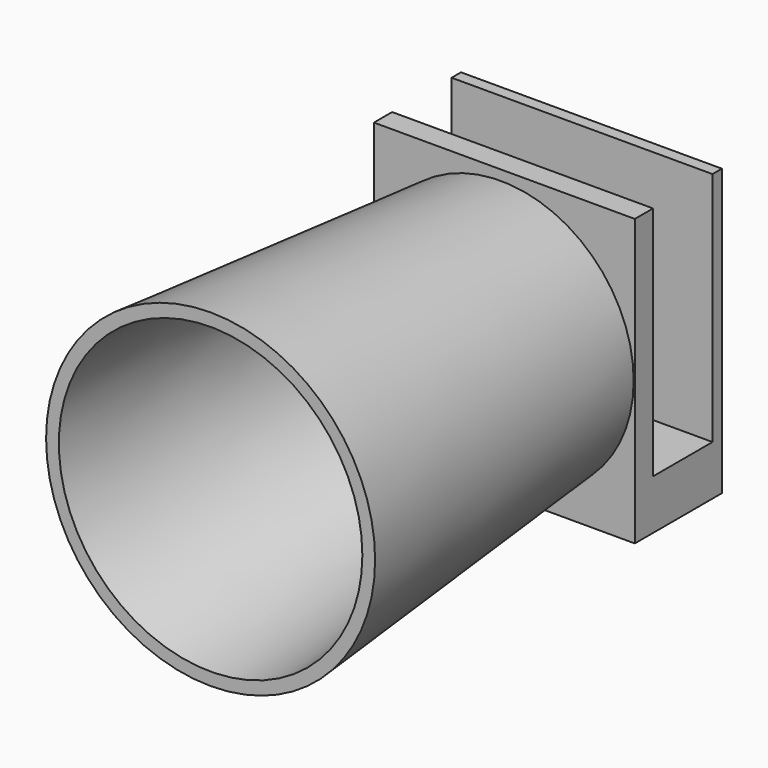
from build123d import *

# Parameters (mm, degrees)
F0_W     = 71.9023197889
F0_H     = 78.7298418581
F1_DEPTH = 30
F2_R     = 36.5885181047
F3_DEPTH = 100
F3_TAPER = -5
F4_T     = -3.5
F5_W     = 71.9023197889
F5_H     = 20.4825603869
F6_DEPTH = 65
F7_R     = 2.9162112623
F8_DEPTH = 0.7


# Not quite as in the source:
# - a feature names something its author has since deleted; it is built from what else it names


with BuildPart() as f1:
    # F0 (on Front) → F1 (new body)
    with BuildSketch(Plane.XZ):
        with Locations((0.9601190686, -0.0165458769)):
            Rectangle(F0_W, F0_H)
    extrude(amount=-F1_DEPTH)

    # F5 (on face) → F6 (cut)
    with BuildSketch(Plane.XY.offset(39.3483750522)):
        with Locations((0.9601190686, 16.5169640677)):
            Rectangle(F5_W, F5_H)
    extrude(amount=-F6_DEPTH, mode=Mode.SUBTRACT)

    # F7 (on face) → F8 (join)
    with BuildSketch(Plane(origin=(0, 0, -39.3814668059), x_dir=(1, 0, 0), z_dir=(0, 0, -1))):
        with BuildLine():
            ThreePointArc((14.4776685496, -14.7840142781), (15.3469177119, -15.6031117856), (16.1666244153, -16.4717864964))
            ThreePointArc((16.1666244153, -16.4717864964), (15.2599699365, -9.1616381984), (8.1129894908, -10.9451630765))
            ThreePointArc((8.1129894908, -10.9451630765), (9.2183727795, -11.3975374989), (10.2953179003, -11.9139714633))
            ThreePointArc((10.2953179003, -11.9139714633), (13.9140775904, -11.1229307961), (14.4776685496, -14.7840142781))
        make_face()
        with BuildLine():
            Line((-21.3132604836, -30), (21.3132604836, -30))
            ThreePointArc((21.3132604836, -30), (19.9831382718, -22.7629352736), (16.1666244153, -16.4717864964))
            ThreePointArc((16.1666244153, -16.4717864964), (15.3469177119, -15.6031117856), (14.4776685496, -14.7840142781))
            ThreePointArc((14.4776685496, -14.7840142781), (12.4762517876, -13.2181928071), (10.2953179003, -11.9139714633))
            ThreePointArc((10.2953179003, -11.9139714633), (9.2183727795, -11.3975374989), (8.1129894908, -10.9451630765))
            ThreePointArc((8.1129894908, -10.9451630765), (4.1215049239, -9.8938814056), (0, -9.6695170536))
            ThreePointArc((0, -9.6695170536), (-4.1215049239, -9.8938814056), (-8.1129894908, -10.9451630765))
            ThreePointArc((-8.1129894908, -10.9451630765), (-9.2183727795, -11.3975374989), (-10.2953179003, -11.9139714633))
            ThreePointArc((-10.2953179003, -11.9139714633), (-12.4762517876, -13.2181928071), (-14.4776685496, -14.7840142781))
            ThreePointArc((-14.4776685496, -14.7840142781), (-15.3469177119, -15.6031117856), (-16.1666244153, -16.4717864964))
            ThreePointArc((-16.1666244153, -16.4717864964), (-19.9831382718, -22.7629352736), (-21.3132604836, -30))
        make_face()
        with BuildLine():
            add(Edge.make_bspline(
                [(0, -23.3312174678), (-0.816430616, -23.1064193373), (-2.3968803534, -23.7472193633), (-1.266410215, -26.0162755449), (-0.3809565691, -26.0923855136), (0, -26.0908510536)],
                knots=[0, 0, 0, 0, 0.3606436386, 0.7173099723, 1, 1, 1, 1], degree=3))
            add(Edge.make_bspline(
                [(0, -23.3312174678), (0.816430616, -23.1064193373), (2.3968803534, -23.7472193633), (1.266410215, -26.0162755449), (0.3809565691, -26.0923855136), (0, -26.0908510536)],
                knots=[0, 0, 0, 0, 0.3606436386, 0.7173099723, 1, 1, 1, 1], degree=3))
        make_face(mode=Mode.SUBTRACT)
        with Locations((-6.3169230707, -18.1775894016)):
            Circle(F7_R, mode=Mode.SUBTRACT)
        with Locations((6.3169230707, -18.1775894016)):
            Circle(F7_R, mode=Mode.SUBTRACT)
        with BuildLine():
            ThreePointArc((-8.1129894908, -10.9451630765), (-15.2599699365, -9.1616381984), (-16.1666244153, -16.4717864964))
            ThreePointArc((-16.1666244153, -16.4717864964), (-15.3469177119, -15.6031117856), (-14.4776685496, -14.7840142781))
            ThreePointArc((-14.4776685496, -14.7840142781), (-13.9140775904, -11.1229307961), (-10.2953179003, -11.9139714633))
            ThreePointArc((-10.2953179003, -11.9139714633), (-9.2183727795, -11.3975374989), (-8.1129894908, -10.9451630765))
        make_face()
    extrude(amount=F8_DEPTH)


with BuildPart() as f3:
    # F2 (on Front) → F3 (new body)
    with BuildSketch(Plane.XZ):
        Circle(F2_R)
    extrude(amount=F3_DEPTH, taper=F3_TAPER)

    # F4
    f4_openings = [f3.faces().sort_by_distance(p)[0] for p in [
        (0, -100, 0),
    ]]
    offset(amount=F4_T, openings=f4_openings, kind=Kind.INTERSECTION)


solid = Compound([f1.part, f3.part])
